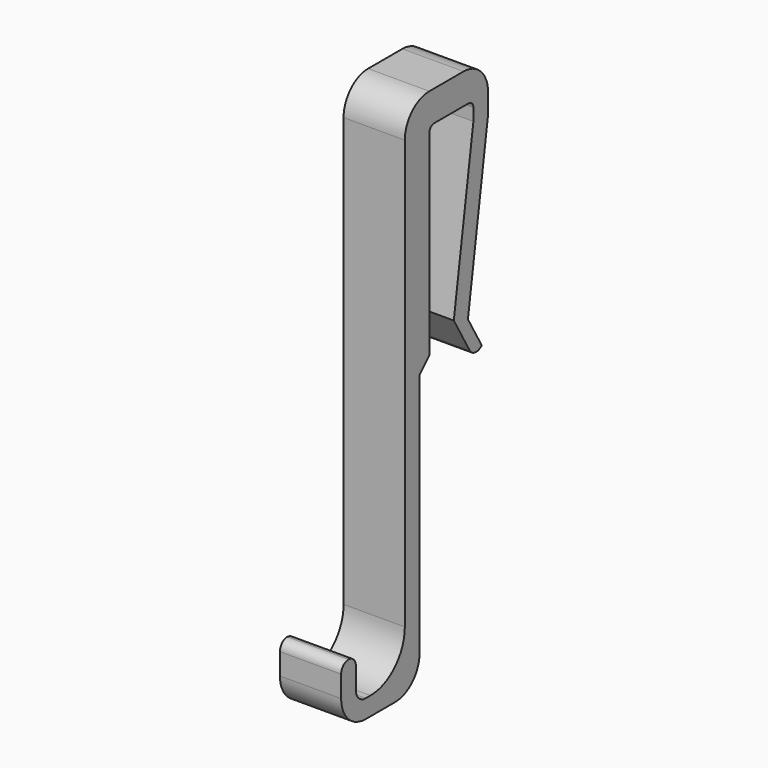
from build123d import *

# Parameters (mm, degrees)
F1_DEPTH = 10
F2_R     = 7
F3_R     = 2
F4_R     = 5
F5_R     = 1.49999
F6_SIZE  = 1.99999
F7_R     = 1


# Not quite as in the source:
# - a fillet or chamfer is up to 0.001 mm smaller than in the source, because OpenCascade refuses the exact size


with BuildPart() as f1:
    # F0 (on Right) → F1 (new body)
    with BuildSketch(Plane.YZ):
        Polygon((0, -35), (0, 0), (9, 0), (9, -3), (5, -30), (9, -36.9282032303), (10.7320508076, -35.9282032303), (7.8850353118, -30.9970277416), (12, -3.2210160959), (12, 5), (-5, 5), (-5, -77), (-15, -77), (-15, -70), (-18, -70), (-18, -80), (-2, -80), (-2, -35), align=None)
    extrude(amount=F1_DEPTH)

    # F2
    f2_edges = [f1.edges().sort_by_distance(p)[0] for p in [
        (5, -5, -77),
    ]]
    fillet(f2_edges, radius=F2_R)

    # F3
    f3_edges = [f1.edges().sort_by_distance(p)[0] for p in [
        (5, -15, -77),
    ]]
    fillet(f3_edges, radius=F3_R)

    # F4
    f4_edges = [f1.edges().sort_by_distance(p)[0] for p in [
        (5, -5, 5),
        (5, 12, 5),
        (5, -18, -80),
        (5, -2, -80),
    ]]
    fillet(f4_edges, radius=F4_R)

    # F5 (radius 1.5 in the source; OpenCascade refuses exactly that, so slightly less here)
    f5_edges = [f1.edges().sort_by_distance(p)[0] for p in [
        (5, 9, -36.928203),
        (5, -18, -70),
        (5, -15, -70),
    ]]
    fillet(f5_edges, radius=F5_R)

    # F6 (size 2 in the source; OpenCascade refuses exactly that, so slightly less here)
    f6_edges = [f1.edges().sort_by_distance(p)[0] for p in [
        (5, 0, -35),
    ]]
    chamfer(f6_edges, length=F6_SIZE)

    # F7
    f7_edges = [f1.edges().sort_by_distance(p)[0] for p in [
        (5, 0, 0),
        (5, 9, 0),
    ]]
    fillet(f7_edges, radius=F7_R)


solid = f1.part
